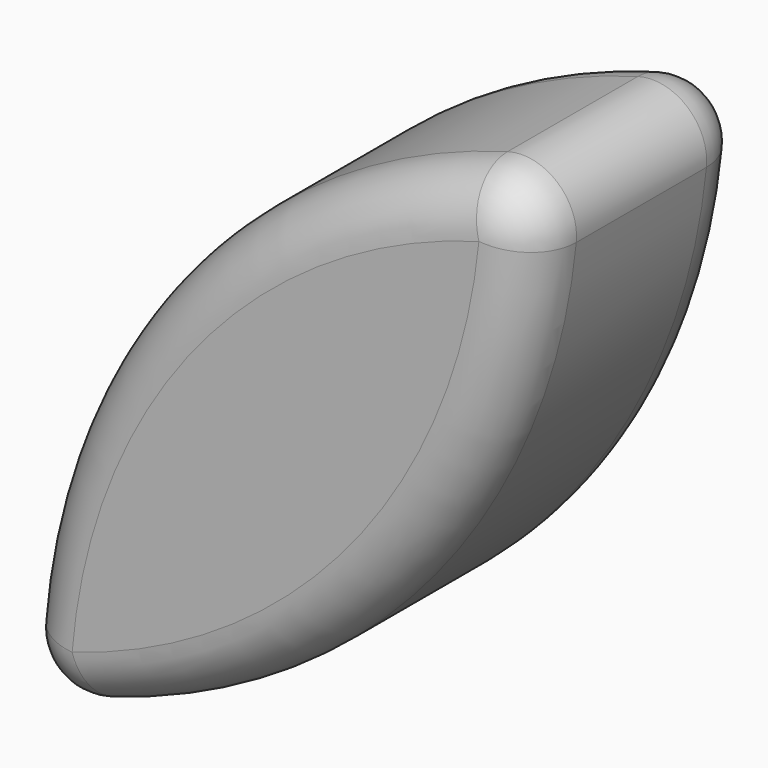
from build123d import *

# Parameters (mm, degrees)
F1_DEPTH = 6.35
F3_R     = 1.27


# Not quite as in the source:
# - a feature of the source that left no trace in its solid (it failed there, or was rolled back) is left out


with BuildPart() as f1:
    # F0 (on Front) → F1 (new body)
    with BuildSketch(Plane.XZ):
        with BuildLine():
            ThreePointArc((0, 0), (8.8014992753, 5.1423850964), (12.1607482433, 14.766623266))
            ThreePointArc((12.1607482433, 14.766623266), (3.270966354, 9.6969414968), (0, 0))
        make_face()
    extrude(amount=F1_DEPTH)

    # F3
    f3_edges = [f1.edges().sort_by_distance(p)[0] for p in [
        (3.270966, 0, 9.696941),
        (8.801499, 0, 5.142385),
        (12.160748, -3.175, 14.766623),
        (0, -3.175, 0),
        (3.270966, -6.35, 9.696941),
        (8.801499, -6.35, 5.142385),
    ]]
    fillet(f3_edges, radius=F3_R)


solid = f1.part
